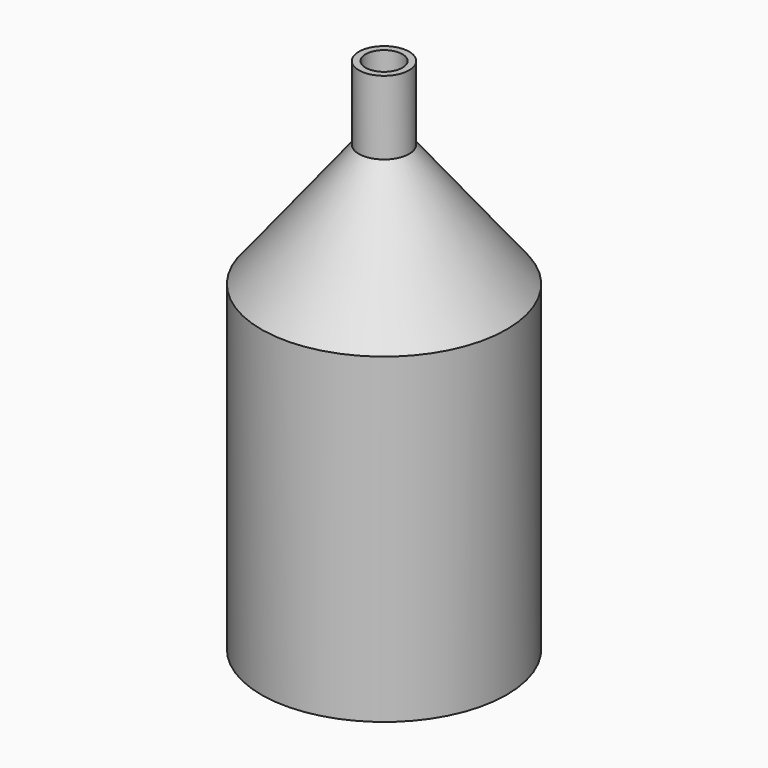
from build123d import *

# Parameters (mm, degrees)
F1_R      = 20
F2_DEPTH  = 1.2
F3_R      = 20
F4_DEPTH  = 1.2
F6_R      = 20
F6_R_2    = 18.8
F7_DEPTH  = 50
F9_R      = 20
F11_R     = 4.1
F13_DEPTH = 12
F15_R     = 3
F16_DEPTH = 25
F14_R     = 18.8


# Not quite as in the source:
# - after a boolean that leaves OpenCascade's solid faulty, fix() repairs it


with BuildPart() as f2:
    # F1 (on Top) → F2 (new body)
    with BuildSketch(Plane.XY):
        Circle(F1_R)
        with BuildLine():
            Line((-18.7904230926, -0.6), (-0.6, -0.6))
            Line((-0.6, -0.6), (-0.6, -18.7904230926))
            ThreePointArc((-0.6, -18.7904230926), (-13.2936074863, -13.2936074863), (-18.7904230926, -0.6))
        make_face(mode=Mode.SUBTRACT)
        with BuildLine():
            Line((0.6, -18.7904230926), (0.6, -0.6))
            Line((0.6, -0.6), (18.7904230926, -0.6))
            ThreePointArc((18.7904230926, -0.6), (13.2936074863, -13.2936074863), (0.6, -18.7904230926))
        make_face(mode=Mode.SUBTRACT)
        with BuildLine():
            Line((-0.6, 18.7904230926), (-0.6, 0.6))
            Line((-0.6, 0.6), (-18.7904230926, 0.6))
            ThreePointArc((-18.7904230926, 0.6), (-13.2936074863, 13.2936074863), (-0.6, 18.7904230926))
        make_face(mode=Mode.SUBTRACT)
        with BuildLine():
            Line((18.7904230926, 0.6), (0.6, 0.6))
            Line((0.6, 0.6), (0.6, 18.7904230926))
            ThreePointArc((0.6, 18.7904230926), (13.2936074863, 13.2936074863), (18.7904230926, 0.6))
        make_face(mode=Mode.SUBTRACT)
    extrude(amount=F2_DEPTH)

    # F3 (on Top) → F4 (join)
    with BuildSketch(Plane.XY):
        Circle(F3_R)
    extrude(amount=-F4_DEPTH)

    # F6 (on offset) → F7 (join)
    with BuildSketch(Plane.XY.offset(1.2)):
        Circle(F6_R)
        Circle(F6_R_2, mode=Mode.SUBTRACT)
    extrude(amount=F7_DEPTH)

    add(f2.part.fix(), mode=Mode.REPLACE)

    # F9 (on offset) → F12 section 0
    with BuildSketch(Plane.XY.offset(51.2)):
        Circle(F9_R)
    # F11 (on offset) → F12 section 1
    with BuildSketch(Plane.XY.offset(71.2)):
        Circle(F11_R)
    loft()

    # F13 (add): a face of the model
    f13_faces = [f2.faces().sort_by_distance(p)[0] for p in [
        (0, 0, 71.2),
    ]]
    extrude(f13_faces, amount=F13_DEPTH)

    # F15 (on offset) → F16 (cut)
    with BuildSketch(Plane.XY.offset(71.2)):
        Circle(F15_R)
    extrude(amount=F16_DEPTH, mode=Mode.SUBTRACT)

    # F14 (on offset) → F17 section 0
    with BuildSketch(Plane.XY.offset(51.2)):
        Circle(F14_R)
    # F15 (on offset) → F17 section 1
    with BuildSketch(Plane.XY.offset(71.2)):
        Circle(F15_R)
    loft(mode=Mode.SUBTRACT)


solid = f2.part
